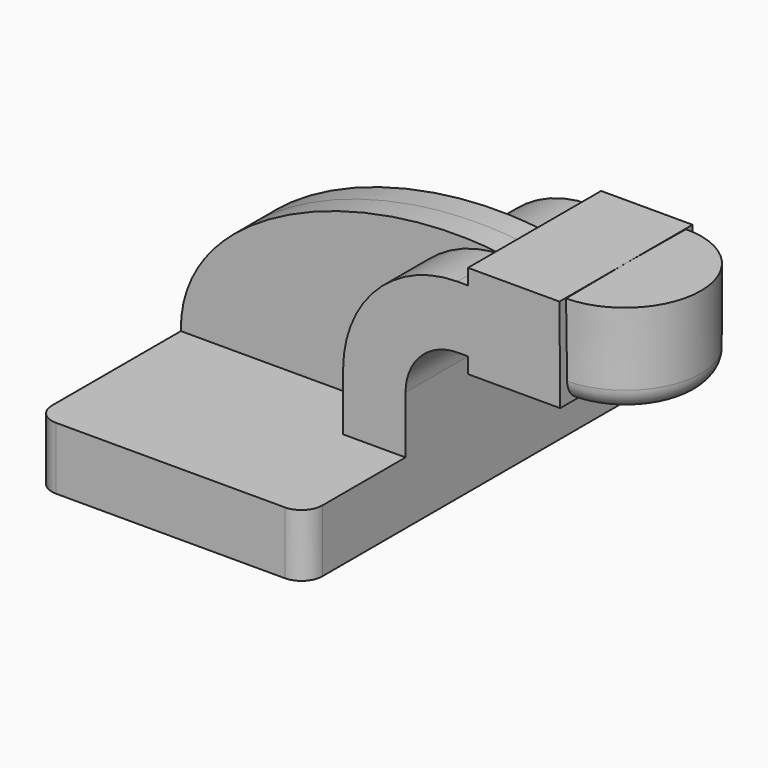
from build123d import *

# Parameters (mm, degrees)
F1_DEPTH    = 63.5
F2_DEPTH    = 25.4
F3_DEPTH    = 7.9375
F5_T1_DEPTH = 50.8


# Not quite as in the source:
# - a fillet or chamfer that OpenCascade refuses, or shapes differently, is made with other operations: its cross-section is extruded or revolved along the edge and cut away or added


with BuildPart() as f1:
    # F0 (on Front) → F1 (new body, symmetric)
    with BuildSketch(Plane.XZ):
        Polygon((22.225, 9.525), (-41.275, 9.525), (-41.275, -9.525), (41.275, -9.525), (41.275, 9.525), align=None)
    extrude(amount=F1_DEPTH, both=True)

    # F0 (on Front) → F2 (join, symmetric)
    with BuildSketch(Plane.XZ):
        with BuildLine():
            Line((22.225, 27.0002), (22.225, 9.525))
            Line((22.225, 9.525), (41.275, 9.525))
            Line((41.275, 9.525), (41.275, 27.0002))
            ThreePointArc((41.275, 27.0002), (45.9246798487, 38.2255201513), (57.15, 42.8752))
            Line((57.15, 42.8752), (60.325, 42.8752))
            Line((60.325, 42.8752), (60.325, 61.9252))
            Line((60.325, 61.9252), (57.15, 61.9252))
            ThreePointArc((57.15, 61.9252), (32.4542956671, 51.6959043329), (22.225, 27.0002))
        make_face()
        Polygon((60.325, 66.675), (60.325, 61.9252), (60.325, 42.8752), (60.325, 38.1), (88.4848684072, 38.1), (88.2495848575, 66.675), align=None)
    extrude(amount=F2_DEPTH, both=True)

    # F0 (on Front) → F3 (join, symmetric)
    with BuildSketch(Plane.XZ):
        with BuildLine():
            add(Edge.make_bspline(
                [(-41.275, 9.525), (-41.8986715376, 44.9499189854), (12.7891246229, 67.7922144532), (57.15, 61.9252)],
                knots=[0, 0, 0, 0, 111.5045361635, 111.5045361635, 111.5045361635, 111.5045361635], degree=3))
            Line((-41.275, 9.525), (22.225, 9.525))
            Line((22.225, 9.525), (22.225, 27.0002))
            ThreePointArc((22.225, 27.0002), (32.4542956671, 51.6959043329), (57.15, 61.9252))
        make_face()
    extrude(amount=F3_DEPTH, both=True)

    # F0 (on Front) → F4 (revolve)
    with BuildSketch(Plane.XZ):
        Polygon((111.125, 66.675), (88.2495848575, 66.675), (88.4848684072, 38.1), (111.125, 38.1), align=None)
    revolve(axis=Axis((88.3672266324, 0, 52.3875), (-0.0082336159, 0, 0.9999661032)))

    # F5: fillet of radius 6.35 on 5 edges, made by hand

    # F5_s2 → F5_t1 (cut)
    with BuildSketch(Plane.XY.offset(-25.4)):
        with BuildLine():
            ThreePointArc((34.925, -63.5), (39.4151280605, -61.6401280605), (41.275, -57.15))
            Line((41.275, -57.15), (41.275, -63.5))
            Line((41.275, -63.5), (34.925, -63.5))
        make_face()
        with BuildLine():
            ThreePointArc((34.925, 63.5), (39.4151280605, 61.6401280605), (41.275, 57.15))
            Line((41.275, 57.15), (41.275, 63.5))
            Line((41.275, 63.5), (34.925, 63.5))
        make_face()
        with BuildLine():
            ThreePointArc((-34.925, 63.5), (-39.4151280605, 61.6401280605), (-41.275, 57.15))
            Line((-41.275, 57.15), (-41.275, 63.5))
            Line((-41.275, 63.5), (-34.925, 63.5))
        make_face()
        with BuildLine():
            ThreePointArc((-34.925, -63.5), (-39.4151280605, -61.6401280605), (-41.275, -57.15))
            Line((-41.275, -57.15), (-41.275, -63.5))
            Line((-41.275, -63.5), (-34.925, -63.5))
        make_face()
    extrude(amount=F5_T1_DEPTH, mode=Mode.SUBTRACT)


with BuildPart() as f5_tool4:
    # F5_s5 → F5_t6 (revolve)
    with BuildSketch(Plane.XZ):
        with BuildLine():
            ThreePointArc((111.125, 44.45), (109.2651280605, 39.9598719395), (104.775, 38.1))
            Line((104.775, 38.1), (111.125, 38.1))
            Line((111.125, 38.1), (111.125, 44.45))
        make_face()
    revolve(axis=Axis((88.4864032368, 0, 37.9135961712), (-0.0082336159, 0, 0.9999661032)))

    split(bisect_by=Plane(origin=(88.7925599353, 0, 0.7311086157), x_dir=(0, 1, 0), z_dir=(0.9999661032, 0, 0.0082336159)), keep=Keep.TOP)

    split(bisect_by=Plane.XY.offset(38.1), keep=Keep.TOP)


with BuildPart() as f1_1:
    add(f1.part)

    # F5_t3: cut F5_tool4
    add(f5_tool4.part, mode=Mode.SUBTRACT)


with BuildPart() as f5_tool10:
    # F5_s11 → F5_t12 (revolve)
    with BuildSketch(Plane.XZ):
        with BuildLine():
            ThreePointArc((111.125, 44.45), (109.2651280605, 39.9598719395), (104.775, 38.1))
            Line((104.775, 38.1), (111.125, 38.1))
            Line((111.125, 38.1), (111.125, 44.45))
        make_face()
    revolve(axis=Axis((88.4864032368, 0, 37.9135961712), (-0.0082336159, 0, 0.9999661032)))

    split(bisect_by=Plane(origin=(88.7925599353, 0, 0.7311086157), x_dir=(0, 1, 0), z_dir=(0.9999661032, 0, 0.0082336159)), keep=Keep.TOP)

    split(bisect_by=Plane.XY.offset(38.1), keep=Keep.BOTTOM)


with BuildPart() as f1_2:
    add(f1_1.part)

    # F5_t9: cut F5_tool10
    add(f5_tool10.part, mode=Mode.SUBTRACT)


with BuildPart() as f5_tool16:
    # F5_s17 → F5_t18 (revolve)
    with BuildSketch(Plane.XZ):
        with BuildLine():
            ThreePointArc((111.125, 44.45), (109.2651280605, 39.9598719395), (104.775, 38.1))
            Line((104.775, 38.1), (111.125, 38.1))
            Line((111.125, 38.1), (111.125, 44.45))
        make_face()
    revolve(axis=Axis((88.4864032368, 0, 37.9135961712), (-0.0082336159, 0, 0.9999661032)))

    split(bisect_by=Plane(origin=(88.7925599353, 0, 0.7311086157), x_dir=(0, 1, 0), z_dir=(-0.9999661032, 0, -0.0082336159)), keep=Keep.TOP)

    split(bisect_by=Plane.XY.offset(38.1), keep=Keep.BOTTOM)


with BuildPart() as f1_3:
    add(f1_2.part)

    # F5_t15: cut F5_tool16
    add(f5_tool16.part, mode=Mode.SUBTRACT)


solid = f1_3.part
